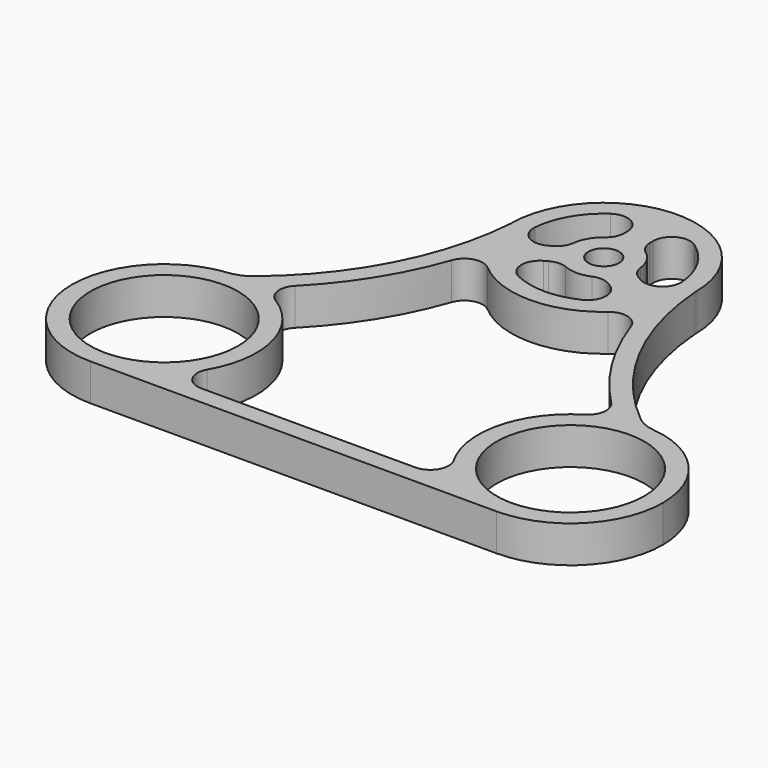
from build123d import *

# Parameters (mm, degrees)
F1_R            = 20
F2_DEPTH        = 10
F3_T            = -5
F4_DEPTH        = 5.001
F1_R_2          = 4.15
F5_DEPTH        = 10
F6_DEPTH        = 10
F6_COPIES_COUNT = 3
F9_R            = 5
F10_T1_DEPTH    = 10
F11_R           = 5


# Not quite as in the source:
# - a fillet or chamfer that OpenCascade refuses, or shapes differently, is made with other operations: its cross-section is extruded or revolved along the edge and cut away or added
# - a feature of the source that left no trace in its solid (it failed there, or was rolled back) is left out
# - a pattern or mirror of a feature is missing from the dataset's text; its kind, count and spacing are read off the source's solid


with BuildPart() as f2:
    # F1 (on Top) → F2 (new body)
    with BuildSketch(Plane.XY):
        with BuildLine():
            ThreePointArc((-25, 0), (0, -25), (25, 0))
            ThreePointArc((25, 0), (0, 25), (-25, 0))
        make_face()
        with BuildLine():
            ThreePointArc((3.5, 19.6913686675), (15.3297097168, 12.8452325787), (20, 0))
            ThreePointArc((20, 0), (-12.8452325787, -15.3297097168), (-3.5, 19.6913686675))
            ThreePointArc((-3.5, 19.6913686675), (0, 20), (3.5, 19.6913686675))
        make_face(mode=Mode.SUBTRACT)
        with BuildLine():
            ThreePointArc((55, -55), (33.982083659, -30.7824998224), (25, 0))
            ThreePointArc((25, 0), (0, -25), (-25, 0))
            ThreePointArc((-25, 0), (-33.982083659, -30.7824998224), (-55, -55))
            ThreePointArc((-55, -55), (-37.3223304703, -62.3223304703), (-30, -80))
            ThreePointArc((-30, -80), (-37.3223304703, -97.6776695297), (-55, -105))
            Line((-55, -105), (55, -105))
            ThreePointArc((55, -105), (30, -80), (55, -55))
        make_face()
        with BuildLine():
            ThreePointArc((80, -80), (72.6776695297, -62.3223304703), (55, -55))
            ThreePointArc((55, -55), (30, -80), (55, -105))
            ThreePointArc((55, -105), (72.6776695297, -97.6776695297), (80, -80))
        make_face()
        with Locations((55, -80)):
            Circle(F1_R, mode=Mode.SUBTRACT)
        with BuildLine():
            ThreePointArc((-30, -80), (-37.3223304703, -62.3223304703), (-55, -55))
            ThreePointArc((-55, -55), (-80, -80), (-55, -105))
            ThreePointArc((-55, -105), (-37.3223304703, -97.6776695297), (-30, -80))
        make_face()
        with Locations((-55, -80)):
            Circle(F1_R, mode=Mode.SUBTRACT)
    extrude(amount=F2_DEPTH)

    # F3
    f3_openings = [f2.faces().sort_by_distance(p)[0] for p in [
        (0, -59.438768, 10),
    ]]
    offset(amount=F3_T, openings=f3_openings)

    # F4 (cut, through all): a face of the model
    f4_faces = [f2.faces().sort_by_distance(p)[0] for p in [
        (0, -60.9945168835, 5),
    ]]
    extrude(f4_faces, amount=-F4_DEPTH, mode=Mode.SUBTRACT)



with BuildPart() as f5:
    # F1 (on Top) → F5 (new body, through all)
    with BuildSketch(Plane.XY):
        with BuildLine():
            ThreePointArc((9.15, 0), (7.6074798718, 5.0841665984), (3.5, 8.4541409972))
            ThreePointArc((3.5, 8.4541409972), (0, 9.15), (-3.5, 8.4541409972))
            ThreePointArc((-3.5, 8.4541409972), (-5.0841665984, -7.6074798718), (9.15, 0))
        make_face()
        Circle(F1_R_2, mode=Mode.SUBTRACT)
    extrude(amount=F5_DEPTH)


with BuildPart() as f2_1:
    add(f2.part)

    add(f5.part)  # F6 merges F5
    # F1 (on Top) → F6 (join, through all)
    with BuildSketch(Plane.XY):
        with BuildLine():
            Line((3.5, 8.4541409972), (3.5, 19.6913686675))
            ThreePointArc((3.5, 19.6913686675), (0, 20), (-3.5, 19.6913686675))
            Line((-3.5, 19.6913686675), (-3.5, 8.4541409972))
            ThreePointArc((-3.5, 8.4541409972), (0, 9.15), (3.5, 8.4541409972))
        make_face()
    f6 = extrude(amount=F6_DEPTH)

    # F6_copies: F6 ×3 about axis
    f6_copies_axis = Axis((0, 0, 0), (0, 0, 1))
    for i in range(1, F6_COPIES_COUNT):
        add(f6.rotate(f6_copies_axis, i * 360 / F6_COPIES_COUNT))

    # F9
    f9_edges = [f2_1.edges().sort_by_distance(p)[0] for p in [
        (3.5, 8.454141, 5),
        (3.5, 19.691369, 5),
        (-3.5, 8.454141, 5),
        (-3.5, 19.691369, 5),
    ]]
    fillet(f9_edges, radius=F9_R)

    # F10: fillet of radius 10 on 4 edges, made by hand

    # F10_s2 → F10_t1 (join)
    with BuildSketch(Plane.XY):
        with BuildLine():
            ThreePointArc((57.6335213289, -55.1390956438), (54.8351268274, -54.4231472749), (52.358111127, -52.9372175751))
            ThreePointArc((52.358111127, -52.9372175751), (53.6675306909, -53.9833691579), (55, -55))
            ThreePointArc((55, -55), (56.3185960515, -55.0347981291), (57.6335213289, -55.1390956438))
        make_face()
        with BuildLine():
            ThreePointArc((-52.358111127, -52.9372175751), (-54.8351268274, -54.4231472749), (-57.6335213289, -55.1390956438))
            ThreePointArc((-57.6335213289, -55.1390956438), (-56.3185960515, -55.0347981291), (-55, -55))
            ThreePointArc((-55, -55), (-53.6675306909, -53.9833691579), (-52.358111127, -52.9372175751))
        make_face()
        with BuildLine():
            ThreePointArc((-24.9985005196, 0.2738097395), (-25.0067330939, -0.0368678872), (-25.0246159735, -0.3471396482))
            ThreePointArc((-25.0246159735, -0.3471396482), (-25.0121066389, -0.1735841019), (-25, 0))
            ThreePointArc((-25, 0), (-24.9996251271, 0.1369069227), (-24.9985005196, 0.2738097395))
        make_face()
        with BuildLine():
            ThreePointArc((24.9985005196, 0.2738097395), (25.0067330939, -0.0368678872), (25.0246159735, -0.3471396482))
            ThreePointArc((25.0246159735, -0.3471396482), (25.0121066389, -0.1735841019), (25, 0))
            ThreePointArc((25, 0), (24.9996251271, 0.1369069227), (24.9985005196, 0.2738097395))
        make_face()
    extrude(amount=F10_T1_DEPTH)

    # F11
    f11_edges = [f2_1.edges().sort_by_distance(p)[0] for p in [
        (9.071501, -1.195982, 5),
        (18.803226, -6.814595, 5),
        (-5.571501, -7.258159, 5),
        (5.571501, -7.258159, 5),
        (15.303226, -12.876773, 5),
        (-15.303226, -12.876773, 5),
        (21.751654, -12.323374, 5),
        (48.164428, -55.952652, 5),
        (40, -100, 5),
        (-40, -100, 5),
        (-48.164428, -55.952652, 5),
        (-21.751654, -12.323374, 5),
        (-9.071501, -1.195982, 5),
        (-18.803226, -6.814595, 5),
    ]]
    fillet(f11_edges, radius=F11_R)


solid = f2_1.part
